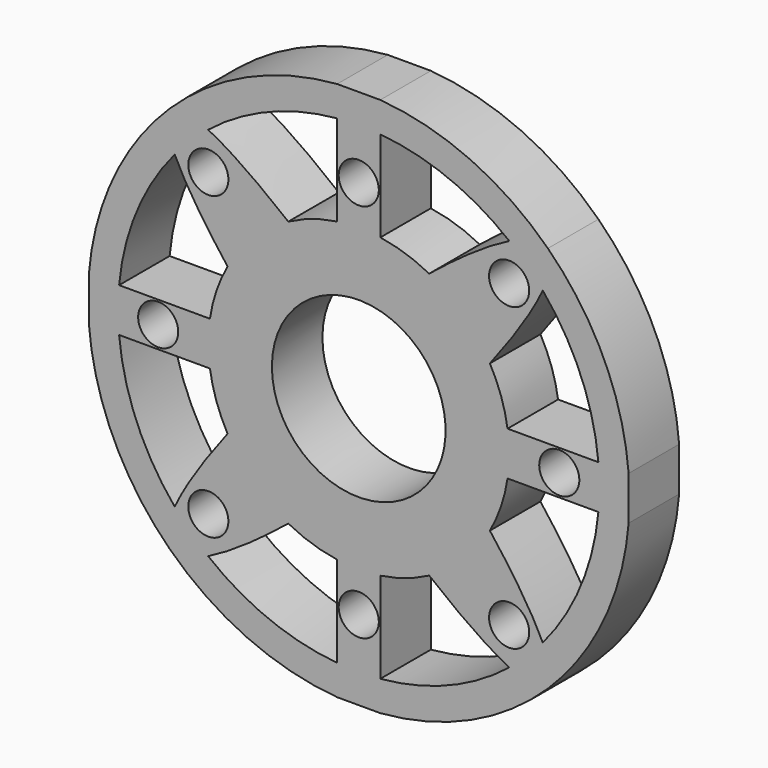
from build123d import *

# Parameters (mm, degrees)
F0_W     = 5.461
F0_H     = 5.5513594167
F1_DEPTH = 8.0000094
F2_D     = 22.0000068
F3_D     = 5.08


# Not quite as in the source:
# - a feature names something its author has since deleted; it is built from what else it names


with BuildPart() as f1:
    # F0 (on Front) → F1 (new body)
    with BuildSketch(Plane.XZ):
        with BuildLine():
            ThreePointArc((18.8467000336, -2.7756797084), (18.9991070269, -1.3915574656), (19.05, 0))
            ThreePointArc((19.05, 0), (18.9991070269, 1.3915574656), (18.8467000336, 2.7756797084))
            Line((18.8467000336, 2.7756797084), (11.213223273, 2.7756797084))
            add(Edge.make_bspline(
                [(8.7331622006, 0), (10.0042735419, 1.3921649666), (11.213223273, 2.7756797084)],
                knots=[1.7496323997, 1.7496323997, 1.7496323997, 1.8611667078, 1.8611667078, 1.8611667078], degree=2, weights=[1, 0.9984454152, 1]))
            add(Edge.make_bspline(
                [(11.213223273, -2.7756797084), (10.0042735419, -1.3921649666), (8.7331622006, 0)],
                knots=[4.4220185994, 4.4220185994, 4.4220185994, 4.5335529075, 4.5335529075, 4.5335529075], degree=2, weights=[1, 0.9984454152, 1]))
            Line((11.213223273, -2.7756797084), (18.8467000336, -2.7756797084))
        make_face()
        with BuildLine():
            ThreePointArc((18.8467000336, 2.7756797084), (18.9991070269, 1.3915574656), (19.05, 0))
            ThreePointArc((19.05, 0), (18.9991070269, -1.3915574656), (18.8467000336, -2.7756797084))
            Line((18.8467000336, -2.7756797084), (30.3533524039, -2.7756797084))
            ThreePointArc((30.3533524039, -2.7756797084), (30.4483216391, -1.3892837594), (30.48, 0))
            ThreePointArc((30.48, 0), (30.4483216391, 1.3892837594), (30.3533524039, 2.7756797084))
            Line((30.3533524039, 2.7756797084), (18.8467000336, 2.7756797084))
        make_face()
        with BuildLine():
            Line((11.213223273, 2.7756797084), (18.8467000336, 2.7756797084))
            ThreePointArc((18.8467000336, 2.7756797084), (18.0293593297, 6.1518047889), (16.612554438, 9.323386458))
            add(Edge.make_bspline(
                [(11.213223273, 2.7756797084), (14.1727224671, 6.1625126409), (16.612554438, 9.323386458)],
                knots=[1.8611667078, 1.8611667078, 1.8611667078, 2.1328025309, 2.1328025309, 2.1328025309], degree=2, weights=[1, 0.9907909168, 1]))
        make_face()
        with BuildLine():
            ThreePointArc((16.612554438, -9.323386458), (18.0293593297, -6.1518047889), (18.8467000336, -2.7756797084))
            Line((18.8467000336, -2.7756797084), (11.213223273, -2.7756797084))
            add(Edge.make_bspline(
                [(16.612554438, -9.323386458), (14.1727224671, -6.1625126409), (11.213223273, -2.7756797084)],
                knots=[4.1503827762, 4.1503827762, 4.1503827762, 4.4220185994, 4.4220185994, 4.4220185994], degree=2, weights=[1, 0.9907909168, 1]))
        make_face()
        with BuildLine():
            add(Edge.make_bspline(
                [(11.213223273, 2.7756797084), (14.1727224671, 6.1625126409), (16.612554438, 9.323386458)],
                knots=[1.8611667078, 1.8611667078, 1.8611667078, 2.1328025309, 2.1328025309, 2.1328025309], degree=2, weights=[1, 0.9907909168, 1]))
            ThreePointArc((16.612554438, 9.323386458), (13.3082399846, 13.6305997121), (8.9231902059, 16.8308994575))
            add(Edge.make_bspline(
                [(8.9231902059, 16.8308994575), (5.928307183, 14.4026430533), (2.7305, 11.4813885374)],
                knots=[4.1503827762, 4.1503827762, 4.1503827762, 4.4127823887, 4.4127823887, 4.4127823887], degree=2, weights=[1, 0.9914056442, 1]))
            Line((2.7305, 11.4813885374), (2.7305, 6.2673374765))
            add(Edge.make_bspline(
                [(6.1445740227, 2.7756797084), (4.4601428488, 4.5445422005), (2.7305, 6.2673374765)],
                knots=[4.6450872157, 4.6450872157, 4.6450872157, 4.7875933171, 4.7875933171, 4.7875933171], degree=2, weights=[1, 0.9974625752, 1]))
            Line((6.1445740227, 2.7756797084), (11.213223273, 2.7756797084))
        make_face()
        with BuildLine():
            ThreePointArc((8.9231902059, 16.8308994575), (13.3082399846, 13.6305997121), (16.612554438, 9.323386458))
            add(Edge.make_bspline(
                [(16.612554438, 9.323386458), (21.3944485628, 15.5184704295), (23.3121649587, 19.6360221261)],
                knots=[2.1328025309, 2.1328025309, 2.1328025309, 2.6562016989, 2.6562016989, 2.6562016989], degree=2, weights=[1, 0.9659516526, 1]))
            ThreePointArc((23.3121649587, 19.6360221261), (21.2931839754, 21.8089595394), (19.0725560053, 23.7753655582))
            add(Edge.make_bspline(
                [(19.0725560053, 23.7753655582), (15.0020729348, 21.759668229), (8.9231902059, 16.8308994575)],
                knots=[3.6269836083, 3.6269836083, 3.6269836083, 4.1503827762, 4.1503827762, 4.1503827762], degree=2, weights=[1, 0.9659516526, 1]))
        make_face()
        with BuildLine():
            add(Edge.make_bspline(
                [(8.7331622006, 0), (10.0042735419, 1.3921649666), (11.213223273, 2.7756797084)],
                knots=[1.7496323997, 1.7496323997, 1.7496323997, 1.8611667078, 1.8611667078, 1.8611667078], degree=2, weights=[1, 0.9984454152, 1]))
            Line((11.213223273, 2.7756797084), (6.1445740227, 2.7756797084))
            add(Edge.make_bspline(
                [(8.7331622006, 0), (7.4620508592, 1.3921649666), (6.1445740227, 2.7756797084)],
                knots=[4.5335529075, 4.5335529075, 4.5335529075, 4.6450872157, 4.6450872157, 4.6450872157], degree=2, weights=[1, 0.9984454152, 1]))
        make_face()
        with BuildLine():
            ThreePointArc((23.3121649587, 19.6360221261), (28.1258728764, 11.745879062), (30.3533524039, 2.7756797084))
            Line((30.3533524039, 2.7756797084), (34.1847616193, 2.7756797084))
            ThreePointArc((34.1847616193, 2.7756797084), (31.0423104315, 14.5834593936), (23.9599066733, 24.5402770362))
            add(Edge.make_bspline(
                [(23.3121649587, 19.6360221261), (25.0847740995, 23.4420123084), (23.9599066733, 24.5402770362)],
                knots=[2.6562016989, 2.6562016989, 2.6562016989, 3.141592646, 3.141592646, 3.141592646], degree=2, weights=[1, 0.9706937258, 1]))
        make_face()
        with BuildLine():
            Line((34.1847616193, 2.7756797084), (30.3533524039, 2.7756797084))
            ThreePointArc((30.3533524039, 2.7756797084), (30.4483216391, 1.3892837594), (30.48, 0))
            ThreePointArc((30.48, 0), (30.4483216391, -1.3892837594), (30.3533524039, -2.7756797084))
            Line((30.3533524039, -2.7756797084), (34.1847616193, -2.7756797084))
            Line((34.1847616193, -2.7756797084), (34.1847616193, 2.7756797084))
        make_face()
        with BuildLine():
            add(Edge.make_bspline(
                [(23.3121649587, -19.6360221261), (21.3944485628, -15.5184704295), (16.612554438, -9.323386458)],
                knots=[3.6269836083, 3.6269836083, 3.6269836083, 4.1503827762, 4.1503827762, 4.1503827762], degree=2, weights=[1, 0.9659516526, 1]))
            ThreePointArc((16.612554438, -9.323386458), (13.3082399846, -13.6305997121), (8.9231902059, -16.8308994575))
            add(Edge.make_bspline(
                [(8.9231902059, -16.8308994575), (15.0020729348, -21.759668229), (19.0725560053, -23.7753655582)],
                knots=[2.1328025309, 2.1328025309, 2.1328025309, 2.6562016989, 2.6562016989, 2.6562016989], degree=2, weights=[1, 0.9659516526, 1]))
            ThreePointArc((19.0725560053, -23.7753655582), (21.2931839754, -21.8089595394), (23.3121649587, -19.6360221261))
        make_face()
        with BuildLine():
            ThreePointArc((8.9231902059, -16.8308994575), (13.3082399846, -13.6305997121), (16.612554438, -9.323386458))
            add(Edge.make_bspline(
                [(16.612554438, -9.323386458), (14.1727224671, -6.1625126409), (11.213223273, -2.7756797084)],
                knots=[4.1503827762, 4.1503827762, 4.1503827762, 4.4220185994, 4.4220185994, 4.4220185994], degree=2, weights=[1, 0.9907909168, 1]))
            Line((11.213223273, -2.7756797084), (6.1445740227, -2.7756797084))
            add(Edge.make_bspline(
                [(2.7305, -6.2673374765), (4.4601428488, -4.5445422005), (6.1445740227, -2.7756797084)],
                knots=[1.4955919901, 1.4955919901, 1.4955919901, 1.6380980915, 1.6380980915, 1.6380980915], degree=2, weights=[1, 0.9974625752, 1]))
            Line((2.7305, -6.2673374765), (2.7305, -11.4813885374))
            add(Edge.make_bspline(
                [(2.7305, -11.4813885374), (5.928307183, -14.4026430533), (8.9231902059, -16.8308994575)],
                knots=[1.8704029185, 1.8704029185, 1.8704029185, 2.1328025309, 2.1328025309, 2.1328025309], degree=2, weights=[1, 0.9914056442, 1]))
        make_face()
        with BuildLine():
            Line((6.1445740227, -2.7756797084), (11.213223273, -2.7756797084))
            add(Edge.make_bspline(
                [(11.213223273, -2.7756797084), (10.0042735419, -1.3921649666), (8.7331622006, 0)],
                knots=[4.4220185994, 4.4220185994, 4.4220185994, 4.5335529075, 4.5335529075, 4.5335529075], degree=2, weights=[1, 0.9984454152, 1]))
            add(Edge.make_bspline(
                [(6.1445740227, -2.7756797084), (7.4620508592, -1.3921649666), (8.7331622006, 0)],
                knots=[1.6380980915, 1.6380980915, 1.6380980915, 1.7496323997, 1.7496323997, 1.7496323997], degree=2, weights=[1, 0.9984454152, 1]))
        make_face()
        with BuildLine():
            Line((34.1847616193, -2.7756797084), (30.3533524039, -2.7756797084))
            ThreePointArc((30.3533524039, -2.7756797084), (28.1258728764, -11.745879062), (23.3121649587, -19.6360221261))
            add(Edge.make_bspline(
                [(23.9599066448, -24.5402770641), (25.0847741234, -23.4420123597), (23.3121649587, -19.6360221261)],
                knots=[3.1415926549, 3.1415926549, 3.1415926549, 3.6269836083, 3.6269836083, 3.6269836083], degree=2, weights=[1, 0.9706937251, 1]))
            ThreePointArc((23.9599066448, -24.5402770641), (31.042310423, -14.5834594117), (34.1847616193, -2.7756797084))
        make_face()
        with BuildLine():
            add(Edge.make_bspline(
                [(8.9231902059, 16.8308994575), (5.928307183, 14.4026430533), (2.7305, 11.4813885374)],
                knots=[4.1503827762, 4.1503827762, 4.1503827762, 4.4127823887, 4.4127823887, 4.4127823887], degree=2, weights=[1, 0.9914056442, 1]))
            ThreePointArc((8.9231902059, 16.8308994575), (5.9139367997, 18.1087783003), (2.7305, 18.8532986437))
            Line((2.7305, 18.8532986437), (2.7305, 11.4813885374))
        make_face()
        with BuildLine():
            ThreePointArc((19.0725560053, 23.7753655582), (21.2931839754, 21.8089595394), (23.3121649587, 19.6360221261))
            add(Edge.make_bspline(
                [(23.3121649587, 19.6360221261), (25.0847740995, 23.4420123084), (23.9599066733, 24.5402770362)],
                knots=[2.6562016989, 2.6562016989, 2.6562016989, 3.141592646, 3.141592646, 3.141592646], degree=2, weights=[1, 0.9706937258, 1]))
            add(Edge.make_bspline(
                [(23.9599066733, 24.5402770362), (22.8350392106, 25.6385417998), (19.0725560053, 23.7753655582)],
                knots=[3.141592646, 3.141592646, 3.141592646, 3.6269836083, 3.6269836083, 3.6269836083], degree=2, weights=[1, 0.970693724, 1]))
        make_face()
        with BuildLine():
            add(Edge.make_bspline(
                [(8.7331622006, 0), (7.4620508592, 1.3921649666), (6.1445740227, 2.7756797084)],
                knots=[4.5335529075, 4.5335529075, 4.5335529075, 4.6450872157, 4.6450872157, 4.6450872157], degree=2, weights=[1, 0.9984454152, 1]))
            Line((6.1445740227, 2.7756797084), (2.7305, 2.7756797084))
            Line((2.7305, 2.7756797084), (2.7305, -2.7756797084))
            Line((2.7305, -2.7756797084), (6.1445740227, -2.7756797084))
            add(Edge.make_bspline(
                [(6.1445740227, -2.7756797084), (7.4620508592, -1.3921649666), (8.7331622006, 0)],
                knots=[1.6380980915, 1.6380980915, 1.6380980915, 1.7496323997, 1.7496323997, 1.7496323997], degree=2, weights=[1, 0.9984454152, 1]))
        make_face()
        with BuildLine():
            Line((2.7305, 2.7756797084), (6.1445740227, 2.7756797084))
            add(Edge.make_bspline(
                [(6.1445740227, 2.7756797084), (4.4601428488, 4.5445422005), (2.7305, 6.2673374765)],
                knots=[4.6450872157, 4.6450872157, 4.6450872157, 4.7875933171, 4.7875933171, 4.7875933171], degree=2, weights=[1, 0.9974625752, 1]))
            Line((2.7305, 6.2673374765), (2.7305, 2.7756797084))
        make_face()
        with BuildLine():
            ThreePointArc((2.7305, -18.8532986437), (5.9139367997, -18.1087783003), (8.9231902059, -16.8308994575))
            add(Edge.make_bspline(
                [(2.7305, -11.4813885374), (5.928307183, -14.4026430533), (8.9231902059, -16.8308994575)],
                knots=[1.8704029185, 1.8704029185, 1.8704029185, 2.1328025309, 2.1328025309, 2.1328025309], degree=2, weights=[1, 0.9914056442, 1]))
            Line((2.7305, -11.4813885374), (2.7305, -18.8532986437))
        make_face()
        with BuildLine():
            add(Edge.make_bspline(
                [(23.9599066448, -24.5402770641), (25.0847741234, -23.4420123597), (23.3121649587, -19.6360221261)],
                knots=[3.1415926549, 3.1415926549, 3.1415926549, 3.6269836083, 3.6269836083, 3.6269836083], degree=2, weights=[1, 0.9706937251, 1]))
            ThreePointArc((23.3121649587, -19.6360221261), (21.2931839754, -21.8089595394), (19.0725560053, -23.7753655582))
            add(Edge.make_bspline(
                [(19.0725560053, -23.7753655582), (22.8350391599, -25.6385417746), (23.9599066448, -24.5402770641)],
                knots=[2.6562016989, 2.6562016989, 2.6562016989, 3.1415926549, 3.1415926549, 3.1415926549], degree=2, weights=[1, 0.9706937248, 1]))
        make_face()
        with BuildLine():
            add(Edge.make_bspline(
                [(2.7305, -6.2673374765), (4.4601428488, -4.5445422005), (6.1445740227, -2.7756797084)],
                knots=[1.4955919901, 1.4955919901, 1.4955919901, 1.6380980915, 1.6380980915, 1.6380980915], degree=2, weights=[1, 0.9974625752, 1]))
            Line((6.1445740227, -2.7756797084), (2.7305, -2.7756797084))
            Line((2.7305, -2.7756797084), (2.7305, -6.2673374765))
        make_face()
        with BuildLine():
            Line((2.7305, 11.4813885374), (2.7305, 18.8532986437))
            ThreePointArc((2.7305, 18.8532986437), (0, 19.05), (-2.7305, 18.8532986437))
            Line((-2.7305, 18.8532986437), (-2.7305, 11.4813885374))
            add(Edge.make_bspline(
                [(0, 8.930517617), (-1.3695558464, 10.2381415163), (-2.7305, 11.4813885374)],
                knots=[4.8997944446, 4.8997944446, 4.8997944446, 5.0119955721, 5.0119955721, 5.0119955721], degree=2, weights=[1, 0.9984267761, 1]))
            add(Edge.make_bspline(
                [(2.7305, 11.4813885374), (1.3695558464, 10.2381415163), (0, 8.930517617)],
                knots=[4.4127823887, 4.4127823887, 4.4127823887, 4.5249835162, 4.5249835162, 4.5249835162], degree=2, weights=[1, 0.9984267761, 1]))
        make_face()
        with BuildLine():
            ThreePointArc((-2.7305, 18.8532986437), (0, 19.05), (2.7305, 18.8532986437))
            Line((2.7305, 18.8532986437), (2.7305, 30.3574499876))
            ThreePointArc((2.7305, 30.3574499876), (0, 30.48), (-2.7305, 30.3574499876))
            Line((-2.7305, 30.3574499876), (-2.7305, 18.8532986437))
        make_face()
        with BuildLine():
            ThreePointArc((2.7305, 30.3574499876), (11.3874611591, 28.2728868061), (19.0725560053, 23.7753655582))
            add(Edge.make_bspline(
                [(23.9599066733, 24.5402770362), (22.8350392106, 25.6385417998), (19.0725560053, 23.7753655582)],
                knots=[3.141592646, 3.141592646, 3.141592646, 3.6269836083, 3.6269836083, 3.6269836083], degree=2, weights=[1, 0.970693724, 1]))
            ThreePointArc((23.9599066733, 24.5402770362), (14.1903495827, 31.2239700156), (2.7305, 34.1884))
            Line((2.7305, 34.1884), (2.7305, 30.3574499876))
        make_face()
        with BuildLine():
            Line((2.7305, 6.2673374765), (2.7305, 11.4813885374))
            add(Edge.make_bspline(
                [(2.7305, 11.4813885374), (1.3695558464, 10.2381415163), (0, 8.930517617)],
                knots=[4.4127823887, 4.4127823887, 4.4127823887, 4.5249835162, 4.5249835162, 4.5249835162], degree=2, weights=[1, 0.9984267761, 1]))
            add(Edge.make_bspline(
                [(2.7305, 6.2673374765), (1.3695558464, 7.6228937178), (0, 8.930517617)],
                knots=[4.7875933171, 4.7875933171, 4.7875933171, 4.8997944446, 4.8997944446, 4.8997944446], degree=2, weights=[1, 0.9984267761, 1]))
        make_face()
        with BuildLine():
            Line((-2.7305, 2.7756797084), (2.7305, 2.7756797084))
            Line((2.7305, 2.7756797084), (2.7305, 6.2673374765))
            add(Edge.make_bspline(
                [(2.7305, 6.2673374765), (1.3695558464, 7.6228937178), (0, 8.930517617)],
                knots=[4.7875933171, 4.7875933171, 4.7875933171, 4.8997944446, 4.8997944446, 4.8997944446], degree=2, weights=[1, 0.9984267761, 1]))
            add(Edge.make_bspline(
                [(0, 8.930517617), (-1.3695558464, 7.6228937178), (-2.7305, 6.2673374765)],
                knots=[4.5249835162, 4.5249835162, 4.5249835162, 4.6371846437, 4.6371846437, 4.6371846437], degree=2, weights=[1, 0.9984267761, 1]))
            Line((-2.7305, 6.2673374765), (-2.7305, 2.7756797084))
        make_face()
        Rectangle(F0_W, F0_H)
        with BuildLine():
            Line((2.7305, -30.3574499876), (2.7305, -18.8532986437))
            ThreePointArc((2.7305, -18.8532986437), (0, -19.05), (-2.7305, -18.8532986437))
            Line((-2.7305, -18.8532986437), (-2.7305, -30.3574499876))
            ThreePointArc((-2.7305, -30.3574499876), (0, -30.48), (2.7305, -30.3574499876))
        make_face()
        with BuildLine():
            ThreePointArc((-2.7305, -18.8532986437), (0, -19.05), (2.7305, -18.8532986437))
            Line((2.7305, -18.8532986437), (2.7305, -11.4813885374))
            add(Edge.make_bspline(
                [(0, -8.930517617), (1.3695558464, -10.2381415163), (2.7305, -11.4813885374)],
                knots=[1.758201791, 1.758201791, 1.758201791, 1.8704029185, 1.8704029185, 1.8704029185], degree=2, weights=[1, 0.9984267761, 1]))
            add(Edge.make_bspline(
                [(-2.7305, -11.4813885374), (-1.3695558464, -10.2381415163), (0, -8.930517617)],
                knots=[1.2711897351, 1.2711897351, 1.2711897351, 1.3833908626, 1.3833908626, 1.3833908626], degree=2, weights=[1, 0.9984267761, 1]))
            Line((-2.7305, -11.4813885374), (-2.7305, -18.8532986437))
        make_face()
        with BuildLine():
            add(Edge.make_bspline(
                [(0, -8.930517617), (1.3695558464, -10.2381415163), (2.7305, -11.4813885374)],
                knots=[1.758201791, 1.758201791, 1.758201791, 1.8704029185, 1.8704029185, 1.8704029185], degree=2, weights=[1, 0.9984267761, 1]))
            Line((2.7305, -11.4813885374), (2.7305, -6.2673374765))
            add(Edge.make_bspline(
                [(0, -8.930517617), (1.3695558464, -7.6228937178), (2.7305, -6.2673374765)],
                knots=[1.3833908626, 1.3833908626, 1.3833908626, 1.4955919901, 1.4955919901, 1.4955919901], degree=2, weights=[1, 0.9984267761, 1]))
        make_face()
        with BuildLine():
            add(Edge.make_bspline(
                [(19.0725560053, -23.7753655582), (22.8350391599, -25.6385417746), (23.9599066448, -24.5402770641)],
                knots=[2.6562016989, 2.6562016989, 2.6562016989, 3.1415926549, 3.1415926549, 3.1415926549], degree=2, weights=[1, 0.9706937248, 1]))
            ThreePointArc((19.0725560053, -23.7753655582), (11.3874611591, -28.2728868061), (2.7305, -30.3574499876))
            Line((2.7305, -30.3574499876), (2.7305, -34.1884))
            ThreePointArc((2.7305, -34.1884), (14.1903495645, -31.2239700238), (23.9599066448, -24.5402770641))
        make_face()
        with BuildLine():
            Line((2.7305, -6.2673374765), (2.7305, -2.7756797084))
            Line((2.7305, -2.7756797084), (-2.7305, -2.7756797084))
            Line((-2.7305, -2.7756797084), (-2.7305, -6.2673374765))
            add(Edge.make_bspline(
                [(-2.7305, -6.2673374765), (-1.3695558464, -7.6228937178), (0, -8.930517617)],
                knots=[1.6460006635, 1.6460006635, 1.6460006635, 1.758201791, 1.758201791, 1.758201791], degree=2, weights=[1, 0.9984267761, 1]))
            add(Edge.make_bspline(
                [(0, -8.930517617), (1.3695558464, -7.6228937178), (2.7305, -6.2673374765)],
                knots=[1.3833908626, 1.3833908626, 1.3833908626, 1.4955919901, 1.4955919901, 1.4955919901], degree=2, weights=[1, 0.9984267761, 1]))
        make_face()
        with BuildLine():
            Line((-2.7305, 11.4813885374), (-2.7305, 18.8532986437))
            ThreePointArc((-2.7305, 18.8532986437), (-5.9139367997, 18.1087783003), (-8.9231902059, 16.8308994575))
            add(Edge.make_bspline(
                [(-2.7305, 11.4813885374), (-5.928307183, 14.4026430533), (-8.9231902059, 16.8308994575)],
                knots=[5.0119955721, 5.0119955721, 5.0119955721, 5.2743951845, 5.2743951845, 5.2743951845], degree=2, weights=[1, 0.9914056442, 1]))
        make_face()
        with BuildLine():
            ThreePointArc((-2.7305, 30.3574499876), (0, 30.48), (2.7305, 30.3574499876))
            Line((2.7305, 30.3574499876), (2.7305, 34.1884))
            Line((2.7305, 34.1884), (-2.7305, 34.1884))
            Line((-2.7305, 34.1884), (-2.7305, 30.3574499876))
        make_face()
        with BuildLine():
            add(Edge.make_bspline(
                [(0, 8.930517617), (-1.3695558464, 7.6228937178), (-2.7305, 6.2673374765)],
                knots=[4.5249835162, 4.5249835162, 4.5249835162, 4.6371846437, 4.6371846437, 4.6371846437], degree=2, weights=[1, 0.9984267761, 1]))
            add(Edge.make_bspline(
                [(0, 8.930517617), (-1.3695558464, 10.2381415163), (-2.7305, 11.4813885374)],
                knots=[4.8997944446, 4.8997944446, 4.8997944446, 5.0119955721, 5.0119955721, 5.0119955721], degree=2, weights=[1, 0.9984267761, 1]))
            Line((-2.7305, 11.4813885374), (-2.7305, 6.2673374765))
        make_face()
        with BuildLine():
            Line((-6.1445740227, 2.7756797084), (-2.7305, 2.7756797084))
            Line((-2.7305, 2.7756797084), (-2.7305, 6.2673374765))
            add(Edge.make_bspline(
                [(-2.7305, 6.2673374765), (-4.4601428488, 4.5445422005), (-6.1445740227, 2.7756797084)],
                knots=[4.6371846437, 4.6371846437, 4.6371846437, 4.7796907451, 4.7796907451, 4.7796907451], degree=2, weights=[1, 0.9974625752, 1]))
        make_face()
        with BuildLine():
            Line((-2.7305, -2.7756797084), (-2.7305, 2.7756797084))
            Line((-2.7305, 2.7756797084), (-6.1445740227, 2.7756797084))
            add(Edge.make_bspline(
                [(-6.1445740227, 2.7756797084), (-7.4620508592, 1.3921649666), (-8.7331622006, 0)],
                knots=[4.7796907451, 4.7796907451, 4.7796907451, 4.8912250533, 4.8912250533, 4.8912250533], degree=2, weights=[1, 0.9984454152, 1]))
            add(Edge.make_bspline(
                [(-8.7331622006, 0), (-7.4620508592, -1.3921649666), (-6.1445740227, -2.7756797084)],
                knots=[1.3919602539, 1.3919602539, 1.3919602539, 1.5034945621, 1.5034945621, 1.5034945621], degree=2, weights=[1, 0.9984454152, 1]))
            Line((-6.1445740227, -2.7756797084), (-2.7305, -2.7756797084))
        make_face()
        with BuildLine():
            ThreePointArc((-8.9231902059, -16.8308994575), (-5.9139367997, -18.1087783003), (-2.7305, -18.8532986437))
            Line((-2.7305, -18.8532986437), (-2.7305, -11.4813885374))
            add(Edge.make_bspline(
                [(-8.9231902059, -16.8308994575), (-5.928307183, -14.4026430533), (-2.7305, -11.4813885374)],
                knots=[1.0087901227, 1.0087901227, 1.0087901227, 1.2711897351, 1.2711897351, 1.2711897351], degree=2, weights=[1, 0.9914056442, 1]))
        make_face()
        with BuildLine():
            Line((2.7305, -34.1884), (2.7305, -30.3574499876))
            ThreePointArc((2.7305, -30.3574499876), (0, -30.48), (-2.7305, -30.3574499876))
            Line((-2.7305, -30.3574499876), (-2.7305, -34.1884))
            Line((-2.7305, -34.1884), (2.7305, -34.1884))
        make_face()
        with BuildLine():
            add(Edge.make_bspline(
                [(-2.7305, -11.4813885374), (-1.3695558464, -10.2381415163), (0, -8.930517617)],
                knots=[1.2711897351, 1.2711897351, 1.2711897351, 1.3833908626, 1.3833908626, 1.3833908626], degree=2, weights=[1, 0.9984267761, 1]))
            add(Edge.make_bspline(
                [(-2.7305, -6.2673374765), (-1.3695558464, -7.6228937178), (0, -8.930517617)],
                knots=[1.6460006635, 1.6460006635, 1.6460006635, 1.758201791, 1.758201791, 1.758201791], degree=2, weights=[1, 0.9984267761, 1]))
            Line((-2.7305, -6.2673374765), (-2.7305, -11.4813885374))
        make_face()
        with BuildLine():
            Line((-2.7305, -6.2673374765), (-2.7305, -2.7756797084))
            Line((-2.7305, -2.7756797084), (-6.1445740227, -2.7756797084))
            add(Edge.make_bspline(
                [(-6.1445740227, -2.7756797084), (-4.4601428488, -4.5445422005), (-2.7305, -6.2673374765)],
                knots=[1.5034945621, 1.5034945621, 1.5034945621, 1.6460006635, 1.6460006635, 1.6460006635], degree=2, weights=[1, 0.9974625752, 1]))
        make_face()
        with BuildLine():
            add(Edge.make_bspline(
                [(-2.7305, 11.4813885374), (-5.928307183, 14.4026430533), (-8.9231902059, 16.8308994575)],
                knots=[5.0119955721, 5.0119955721, 5.0119955721, 5.2743951845, 5.2743951845, 5.2743951845], degree=2, weights=[1, 0.9914056442, 1]))
            ThreePointArc((-8.9231902059, 16.8308994575), (-13.3082399846, 13.6305997121), (-16.612554438, 9.323386458))
            add(Edge.make_bspline(
                [(-16.612554438, 9.323386458), (-14.1727224671, 6.1625126409), (-11.213223273, 2.7756797084)],
                knots=[1.0087901227, 1.0087901227, 1.0087901227, 1.2804259458, 1.2804259458, 1.2804259458], degree=2, weights=[1, 0.9907909168, 1]))
            Line((-11.213223273, 2.7756797084), (-6.1445740227, 2.7756797084))
            add(Edge.make_bspline(
                [(-2.7305, 6.2673374765), (-4.4601428488, 4.5445422005), (-6.1445740227, 2.7756797084)],
                knots=[4.6371846437, 4.6371846437, 4.6371846437, 4.7796907451, 4.7796907451, 4.7796907451], degree=2, weights=[1, 0.9974625752, 1]))
            Line((-2.7305, 6.2673374765), (-2.7305, 11.4813885374))
        make_face()
        with BuildLine():
            ThreePointArc((-16.612554438, 9.323386458), (-13.3082399846, 13.6305997121), (-8.9231902059, 16.8308994575))
            add(Edge.make_bspline(
                [(-8.9231902059, 16.8308994575), (-15.0020729348, 21.759668229), (-19.0725560053, 23.7753655582)],
                knots=[5.2743951845, 5.2743951845, 5.2743951845, 5.7977943525, 5.7977943525, 5.7977943525], degree=2, weights=[1, 0.9659516526, 1]))
            ThreePointArc((-19.0725560053, 23.7753655582), (-21.2931839754, 21.8089595394), (-23.3121649587, 19.6360221261))
            add(Edge.make_bspline(
                [(-23.3121649587, 19.6360221261), (-21.3944485628, 15.5184704295), (-16.612554438, 9.323386458)],
                knots=[0.4853909547, 0.4853909547, 0.4853909547, 1.0087901227, 1.0087901227, 1.0087901227], degree=2, weights=[1, 0.9659516526, 1]))
        make_face()
        with BuildLine():
            ThreePointArc((-19.0725560053, 23.7753655582), (-11.3874611591, 28.2728868061), (-2.7305, 30.3574499876))
            Line((-2.7305, 30.3574499876), (-2.7305, 34.1884))
            ThreePointArc((-2.7305, 34.1884), (-14.1903495608, 31.2239700255), (-23.9599066389, 24.5402770698))
            add(Edge.make_bspline(
                [(-19.0725560053, 23.7753655582), (-22.8350391496, 25.6385417695), (-23.9599066389, 24.5402770698)],
                knots=[5.7977943525, 5.7977943525, 5.7977943525, 6.2831853072, 6.2831853072, 6.2831853072], degree=2, weights=[1, 0.9706937249, 1]))
        make_face()
        with BuildLine():
            add(Edge.make_bspline(
                [(-6.1445740227, 2.7756797084), (-7.4620508592, 1.3921649666), (-8.7331622006, 0)],
                knots=[4.7796907451, 4.7796907451, 4.7796907451, 4.8912250533, 4.8912250533, 4.8912250533], degree=2, weights=[1, 0.9984454152, 1]))
            Line((-6.1445740227, 2.7756797084), (-11.213223273, 2.7756797084))
            add(Edge.make_bspline(
                [(-11.213223273, 2.7756797084), (-10.0042735419, 1.3921649666), (-8.7331622006, 0)],
                knots=[1.2804259458, 1.2804259458, 1.2804259458, 1.3919602539, 1.3919602539, 1.3919602539], degree=2, weights=[1, 0.9984454152, 1]))
        make_face()
        with BuildLine():
            add(Edge.make_bspline(
                [(-19.0725560053, -23.7753655582), (-15.0020729348, -21.759668229), (-8.9231902059, -16.8308994575)],
                knots=[0.4853909547, 0.4853909547, 0.4853909547, 1.0087901227, 1.0087901227, 1.0087901227], degree=2, weights=[1, 0.9659516526, 1]))
            ThreePointArc((-8.9231902059, -16.8308994575), (-13.3082399846, -13.6305997121), (-16.612554438, -9.323386458))
            add(Edge.make_bspline(
                [(-16.612554438, -9.323386458), (-21.3944485628, -15.5184704295), (-23.3121649587, -19.6360221261)],
                knots=[5.2743951845, 5.2743951845, 5.2743951845, 5.7977943525, 5.7977943525, 5.7977943525], degree=2, weights=[1, 0.9659516526, 1]))
            ThreePointArc((-23.3121649587, -19.6360221261), (-21.2931839754, -21.8089595394), (-19.0725560053, -23.7753655582))
        make_face()
        with BuildLine():
            ThreePointArc((-16.612554438, -9.323386458), (-13.3082399846, -13.6305997121), (-8.9231902059, -16.8308994575))
            add(Edge.make_bspline(
                [(-8.9231902059, -16.8308994575), (-5.928307183, -14.4026430533), (-2.7305, -11.4813885374)],
                knots=[1.0087901227, 1.0087901227, 1.0087901227, 1.2711897351, 1.2711897351, 1.2711897351], degree=2, weights=[1, 0.9914056442, 1]))
            Line((-2.7305, -11.4813885374), (-2.7305, -6.2673374765))
            add(Edge.make_bspline(
                [(-6.1445740227, -2.7756797084), (-4.4601428488, -4.5445422005), (-2.7305, -6.2673374765)],
                knots=[1.5034945621, 1.5034945621, 1.5034945621, 1.6460006635, 1.6460006635, 1.6460006635], degree=2, weights=[1, 0.9974625752, 1]))
            Line((-6.1445740227, -2.7756797084), (-11.213223273, -2.7756797084))
            add(Edge.make_bspline(
                [(-11.213223273, -2.7756797084), (-14.1727224671, -6.1625126409), (-16.612554438, -9.323386458)],
                knots=[5.0027593614, 5.0027593614, 5.0027593614, 5.2743951845, 5.2743951845, 5.2743951845], degree=2, weights=[1, 0.9907909168, 1]))
        make_face()
        with BuildLine():
            Line((-2.7305, -34.1884), (-2.7305, -30.3574499876))
            ThreePointArc((-2.7305, -30.3574499876), (-11.3874611591, -28.2728868061), (-19.0725560053, -23.7753655582))
            add(Edge.make_bspline(
                [(-23.9599066389, -24.5402770698), (-22.8350391496, -25.6385417695), (-19.0725560053, -23.7753655582)],
                knots=[0, 0, 0, 0.4853909547, 0.4853909547, 0.4853909547], degree=2, weights=[1, 0.9706937249, 1]))
            ThreePointArc((-23.9599066389, -24.5402770698), (-14.1903495608, -31.2239700255), (-2.7305, -34.1884))
        make_face()
        with BuildLine():
            Line((-11.213223273, -2.7756797084), (-6.1445740227, -2.7756797084))
            add(Edge.make_bspline(
                [(-8.7331622006, 0), (-7.4620508592, -1.3921649666), (-6.1445740227, -2.7756797084)],
                knots=[1.3919602539, 1.3919602539, 1.3919602539, 1.5034945621, 1.5034945621, 1.5034945621], degree=2, weights=[1, 0.9984454152, 1]))
            add(Edge.make_bspline(
                [(-8.7331622006, 0), (-10.0042735419, -1.3921649666), (-11.213223273, -2.7756797084)],
                knots=[4.8912250533, 4.8912250533, 4.8912250533, 5.0027593614, 5.0027593614, 5.0027593614], degree=2, weights=[1, 0.9984454152, 1]))
        make_face()
        with BuildLine():
            add(Edge.make_bspline(
                [(-16.612554438, 9.323386458), (-14.1727224671, 6.1625126409), (-11.213223273, 2.7756797084)],
                knots=[1.0087901227, 1.0087901227, 1.0087901227, 1.2804259458, 1.2804259458, 1.2804259458], degree=2, weights=[1, 0.9907909168, 1]))
            ThreePointArc((-16.612554438, 9.323386458), (-18.0293593297, 6.1518047889), (-18.8467000336, 2.7756797084))
            Line((-18.8467000336, 2.7756797084), (-11.213223273, 2.7756797084))
        make_face()
        with BuildLine():
            ThreePointArc((-23.3121649587, 19.6360221261), (-21.2931839754, 21.8089595394), (-19.0725560053, 23.7753655582))
            add(Edge.make_bspline(
                [(-19.0725560053, 23.7753655582), (-22.8350391496, 25.6385417695), (-23.9599066389, 24.5402770698)],
                knots=[5.7977943525, 5.7977943525, 5.7977943525, 6.2831853072, 6.2831853072, 6.2831853072], degree=2, weights=[1, 0.9706937249, 1]))
            add(Edge.make_bspline(
                [(-23.9599066389, 24.5402770698), (-25.0847741283, 23.4420123701), (-23.3121649587, 19.6360221261)],
                knots=[0, 0, 0, 0.4853909547, 0.4853909547, 0.4853909547], degree=2, weights=[1, 0.9706937249, 1]))
        make_face()
        with BuildLine():
            add(Edge.make_bspline(
                [(-23.9599066389, 24.5402770698), (-25.0847741283, 23.4420123701), (-23.3121649587, 19.6360221261)],
                knots=[0, 0, 0, 0.4853909547, 0.4853909547, 0.4853909547], degree=2, weights=[1, 0.9706937249, 1]))
            ThreePointArc((-23.9599066389, 24.5402770698), (-31.0423104213, 14.5834594154), (-34.1847616193, 2.7756797084))
            Line((-34.1847616193, 2.7756797084), (-30.3533524039, 2.7756797084))
            ThreePointArc((-30.3533524039, 2.7756797084), (-28.1258728764, 11.745879062), (-23.3121649587, 19.6360221261))
        make_face()
        with BuildLine():
            add(Edge.make_bspline(
                [(-11.213223273, 2.7756797084), (-10.0042735419, 1.3921649666), (-8.7331622006, 0)],
                knots=[1.2804259458, 1.2804259458, 1.2804259458, 1.3919602539, 1.3919602539, 1.3919602539], degree=2, weights=[1, 0.9984454152, 1]))
            Line((-11.213223273, 2.7756797084), (-18.8467000336, 2.7756797084))
            ThreePointArc((-18.8467000336, 2.7756797084), (-19.05, 0), (-18.8467000336, -2.7756797084))
            Line((-18.8467000336, -2.7756797084), (-11.213223273, -2.7756797084))
            add(Edge.make_bspline(
                [(-8.7331622006, 0), (-10.0042735419, -1.3921649666), (-11.213223273, -2.7756797084)],
                knots=[4.8912250533, 4.8912250533, 4.8912250533, 5.0027593614, 5.0027593614, 5.0027593614], degree=2, weights=[1, 0.9984454152, 1]))
        make_face()
        with BuildLine():
            ThreePointArc((-18.8467000336, -2.7756797084), (-18.0293593297, -6.1518047889), (-16.612554438, -9.323386458))
            add(Edge.make_bspline(
                [(-11.213223273, -2.7756797084), (-14.1727224671, -6.1625126409), (-16.612554438, -9.323386458)],
                knots=[5.0027593614, 5.0027593614, 5.0027593614, 5.2743951845, 5.2743951845, 5.2743951845], degree=2, weights=[1, 0.9907909168, 1]))
            Line((-11.213223273, -2.7756797084), (-18.8467000336, -2.7756797084))
        make_face()
        with BuildLine():
            add(Edge.make_bspline(
                [(-23.9599066389, -24.5402770698), (-22.8350391496, -25.6385417695), (-19.0725560053, -23.7753655582)],
                knots=[0, 0, 0, 0.4853909547, 0.4853909547, 0.4853909547], degree=2, weights=[1, 0.9706937249, 1]))
            ThreePointArc((-19.0725560053, -23.7753655582), (-21.2931839754, -21.8089595394), (-23.3121649587, -19.6360221261))
            add(Edge.make_bspline(
                [(-23.3121649587, -19.6360221261), (-25.0847741283, -23.4420123701), (-23.9599066389, -24.5402770698)],
                knots=[5.7977943525, 5.7977943525, 5.7977943525, 6.2831853072, 6.2831853072, 6.2831853072], degree=2, weights=[1, 0.9706937249, 1]))
        make_face()
        with BuildLine():
            ThreePointArc((-34.1847616193, -2.7756797084), (-31.0423104213, -14.5834594154), (-23.9599066389, -24.5402770698))
            add(Edge.make_bspline(
                [(-23.3121649587, -19.6360221261), (-25.0847741283, -23.4420123701), (-23.9599066389, -24.5402770698)],
                knots=[5.7977943525, 5.7977943525, 5.7977943525, 6.2831853072, 6.2831853072, 6.2831853072], degree=2, weights=[1, 0.9706937249, 1]))
            ThreePointArc((-23.3121649587, -19.6360221261), (-28.1258728764, -11.745879062), (-30.3533524039, -2.7756797084))
            Line((-30.3533524039, -2.7756797084), (-34.1847616193, -2.7756797084))
        make_face()
        with BuildLine():
            ThreePointArc((-18.8467000336, -2.7756797084), (-19.05, 0), (-18.8467000336, 2.7756797084))
            Line((-18.8467000336, 2.7756797084), (-30.3533524039, 2.7756797084))
            ThreePointArc((-30.3533524039, 2.7756797084), (-30.48, 0), (-30.3533524039, -2.7756797084))
            Line((-30.3533524039, -2.7756797084), (-18.8467000336, -2.7756797084))
        make_face()
        with BuildLine():
            Line((-30.3533524039, 2.7756797084), (-34.1847616193, 2.7756797084))
            Line((-34.1847616193, 2.7756797084), (-34.1847616193, -2.7756797084))
            Line((-34.1847616193, -2.7756797084), (-30.3533524039, -2.7756797084))
            ThreePointArc((-30.3533524039, -2.7756797084), (-30.48, 0), (-30.3533524039, 2.7756797084))
        make_face()
    extrude(amount=F1_DEPTH)

    # F2 (through all)
    with Locations(Plane(origin=(0, 0, 0), x_dir=(1, 0, 0), z_dir=(0, 1, 0))):
        with Locations((0, 0)):
            Hole(F2_D / 2)

    # F3 (through all)
    with Locations(Plane(origin=(0, 0, 0), x_dir=(1, 0, 0), z_dir=(0, 1, 0))):
        with Locations((-25.4, 0), (0, -24.0799499585), (25.4, 0), (0, 24.0799499585), (-19.05, -19.05), (19.05, -19.05), (19.05, 19.05), (-19.05, 19.05)):
            Hole(F3_D / 2)


solid = f1.part
